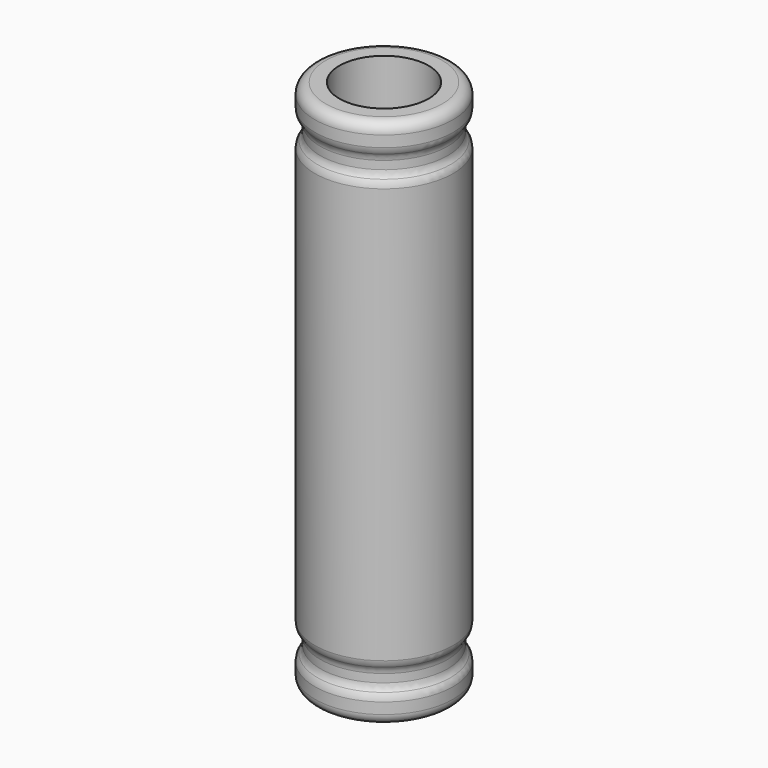
from build123d import *

# Parameters (mm, degrees)
F0_R     = 16.51
F0_R_2   = 10.668
F1_DEPTH = 127
F3_R     = 16.9570806309
F3_R_2   = 15.24
F4_DEPTH = 6.35
F6_R     = 19.4483101308
F6_R_2   = 15.24
F7_DEPTH = 6.35
F8_R     = 2.54
F11_R    = 2.54
F14_R    = 2.54


# Not quite as in the source:
# - a fillet or chamfer that OpenCascade refuses, or shapes differently, is made with other operations: its cross-section is extruded or revolved along the edge and cut away or added


with BuildPart() as f1:
    # F0 (on Top) → F1 (new body)
    with BuildSketch(Plane.XY):
        Circle(F0_R)
        Circle(F0_R_2, mode=Mode.SUBTRACT)
    extrude(amount=F1_DEPTH)

    # F3 (on offset) → F4 (cut)
    with BuildSketch(Plane.XY.offset(114.3)):
        Circle(F3_R)
        Circle(F3_R_2, mode=Mode.SUBTRACT)
    extrude(amount=F4_DEPTH, mode=Mode.SUBTRACT)

    # F6 (on offset) → F7 (cut)
    with BuildSketch(Plane(origin=(0, 0, 12.7), x_dir=(1, 0, 0), z_dir=(0, 0, -1))):
        Circle(F6_R)
        Circle(F6_R_2, mode=Mode.SUBTRACT)
    extrude(amount=F7_DEPTH, mode=Mode.SUBTRACT)

    # F8
    f8_edges = [f1.edges().sort_by_distance(p)[0] for p in [
        (-16.51, 0, 0),
    ]]
    fillet(f8_edges, radius=F8_R)

    # F9: fillet of radius 2.54 on 1 edges, made by hand

    # F9_s1 → F9_t2 (revolve)
    with BuildSketch(Plane.XZ):
        with BuildLine():
            ThreePointArc((15.24, 10.5002954744), (15.5802954744, 11.7702954744), (16.51, 12.7))
            Line((16.51, 12.7), (15.24, 12.7))
            Line((15.24, 12.7), (15.24, 10.5002954744))
        make_face()
    revolve(axis=Axis((0, 0, 12.7), (0, 0, -1)))

    # F10: fillet of radius 2.54 on 1 edges, made by hand

    # F10_s1 → F10_t2 (revolve)
    with BuildSketch(Plane.XZ):
        with BuildLine():
            ThreePointArc((16.51, 6.35), (15.5802954744, 7.2797045256), (15.24, 8.5497045256))
            Line((15.24, 8.5497045256), (15.24, 6.35))
            Line((15.24, 6.35), (16.51, 6.35))
        make_face()
    revolve(axis=Axis((0, 0, 6.35), (0, 0, -1)))

    # F11
    f11_edges = [f1.edges().sort_by_distance(p)[0] for p in [
        (-16.51, 0, 12.7),
        (-16.51, 0, 6.35),
    ]]
    fillet(f11_edges, radius=F11_R)

    # F12: fillet of radius 2.54 on 2 edges, made by hand

    # F12_s1 → F12_t2 (revolve)
    with BuildSketch(Plane.XZ):
        with BuildLine():
            ThreePointArc((16.51, 114.3), (15.5802954744, 115.2297045256), (15.24, 116.4997045256))
            Line((15.24, 116.4997045256), (15.24, 114.3))
            Line((15.24, 114.3), (16.51, 114.3))
        make_face()
    revolve(axis=Axis((0, 0, 114.3), (0, 0, 1)))

    # F12_s3 → F12_t4 (revolve, cut)
    with BuildSketch(Plane.XZ):
        with BuildLine():
            ThreePointArc((13.97, 127), (15.7660512242, 126.2560512242), (16.51, 124.46))
            Line((16.51, 124.46), (16.51, 127))
            Line((16.51, 127), (13.97, 127))
        make_face()
    revolve(axis=Axis((0, 0, 127), (0, 0, 1)), mode=Mode.SUBTRACT)

    # F13: fillet of radius 2.54 on 1 edges, made by hand

    # F13_s1 → F13_t2 (revolve)
    with BuildSketch(Plane.XZ):
        with BuildLine():
            ThreePointArc((16.51, 120.65), (15.5802954744, 119.7202954744), (15.24, 118.4502954744))
            Line((15.24, 118.4502954744), (15.24, 120.65))
            Line((15.24, 120.65), (16.51, 120.65))
        make_face()
    revolve(axis=Axis((0, 0, 120.65), (0, 0, 1)))

    # F14
    f14_edges = [f1.edges().sort_by_distance(p)[0] for p in [
        (-16.51, 0, 120.65),
        (-16.51, 0, 114.3),
    ]]
    fillet(f14_edges, radius=F14_R)


solid = f1.part
